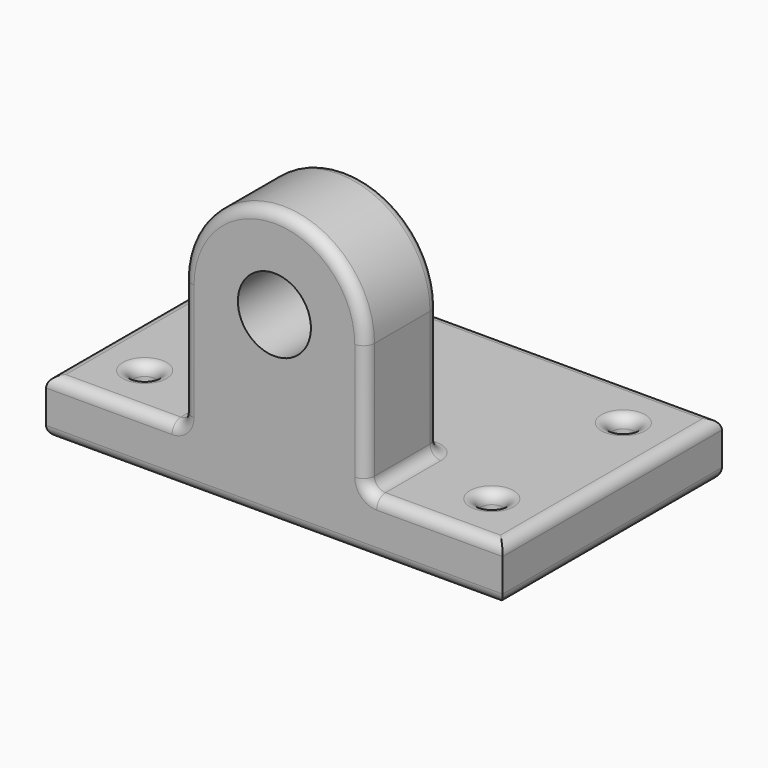
from build123d import *

# Parameters (mm, degrees)
F0_W     = 125
F0_H     = 75
F1_DEPTH = 15
F3_DEPTH = 25
F4_R     = 3
F5_DEPTH = 15
F6_R     = 3


with BuildPart() as f1:
    # F0 (on Top) → F1 (new body)
    with BuildSketch(Plane.XY):
        Rectangle(F0_W, F0_H)
    extrude(amount=F1_DEPTH)

    # F2 (on face) → F3 (join)
    with BuildSketch(Plane.XZ.offset(37.5)):
        with BuildLine():
            Line((10, 50), (25, 50))
            ThreePointArc((25, 50), (0, 75), (-25, 50))
            Line((-25, 50), (-10, 50))
            ThreePointArc((-10, 50), (0, 60), (10, 50))
        make_face()
        with BuildLine():
            Line((-25, 15), (25, 15))
            Line((25, 15), (25, 50))
            ThreePointArc((25, 50), (0, 25), (-25, 50))
            Line((-25, 50), (-25, 15))
        make_face()
        with BuildLine():
            ThreePointArc((-25, 50), (0, 25), (25, 50))
            Line((25, 50), (10, 50))
            ThreePointArc((10, 50), (0, 40), (-10, 50))
            Line((-10, 50), (-25, 50))
        make_face()
    extrude(amount=-F3_DEPTH)

    # F4 (on face) → F5 (cut, through all)
    with BuildSketch(Plane.XY.offset(15)):
        with Locations((-47.5, -22.5)):
            Circle(F4_R)
        with Locations((47.5, 22.5)):
            Circle(F4_R)
        with Locations((47.5, -22.5)):
            Circle(F4_R)
        with Locations((-47.5, 22.5)):
            Circle(F4_R)
    extrude(amount=-F5_DEPTH, mode=Mode.SUBTRACT)

    # F6
    f6_edges = [f1.edges().sort_by_distance(p)[0] for p in [
        (43.75, -37.5, 15),
        (25, -25, 15),
        (62.5, 0, 15),
        (0, -12.5, 15),
        (0, 37.5, 15),
        (-25, -25, 15),
        (-62.5, 0, 15),
        (-43.75, -37.5, 15),
        (-50.5, -22.5, 15),
        (44.5, -22.5, 15),
        (-50.5, 22.5, 15),
        (44.5, 22.5, 15),
        (-10, -12.5, 50),
        (0, -12.5, 75),
        (-25, -12.5, 32.5),
        (25, -12.5, 32.5),
        (62.5, 0, 0),
        (0, -37.5, 0),
        (0, 37.5, 0),
        (-62.5, 0, 0),
        (-50.5, -22.5, 0),
        (44.5, -22.5, 0),
        (-50.5, 22.5, 0),
        (44.5, 22.5, 0),
        (-25, -37.5, 32.5),
        (0, -37.5, 75),
        (25, -37.5, 32.5),
    ]]
    fillet(f6_edges, radius=F6_R)


solid = f1.part
